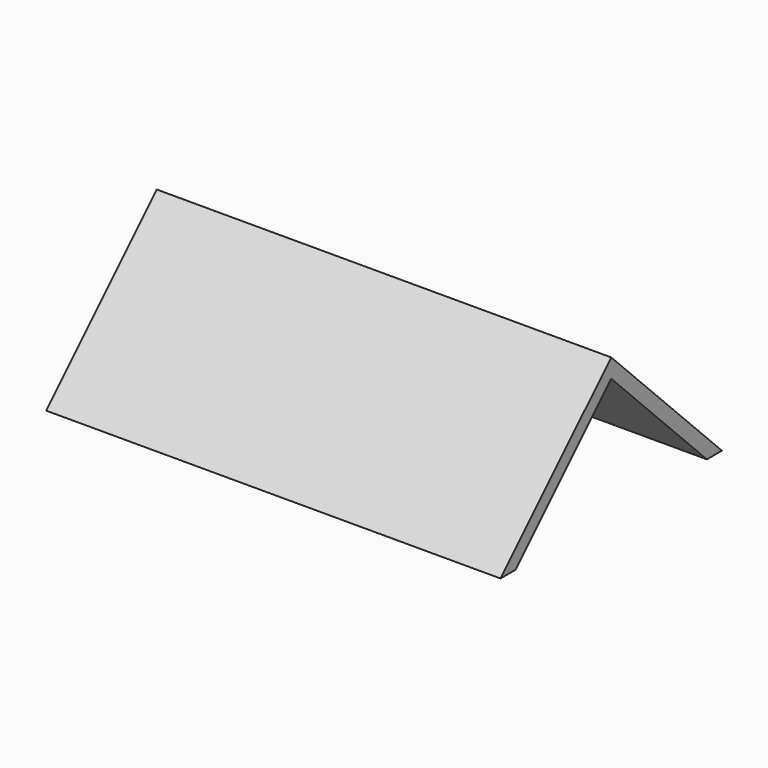
from build123d import *

# Parameters (mm, degrees)
F1_DEPTH = 60
F2_DEPTH = 8.4


with BuildPart() as f1:
    # F0 (on Right) → F1 (new body)
    with BuildSketch(Plane.YZ):
        Polygon((-124.5425649285, 38.5748143829), (-106.5425649285, 56.5748143829), (-88.5425649285, 38.5748143829), (-85.7141378038, 38.5748143829), (-87.1283513662, 39.9890279453), (-106.5425649285, 59.4032415077), (-125.9567784909, 39.9890279453), (-127.3709920533, 38.5748143829), align=None)
    extrude(amount=F1_DEPTH)

    # F2 (add): a face of the model
    f2_faces = [f1.faces().sort_by_distance(p)[0] for p in [
        (0, -125.9567784909, 39.0405521721),
    ]]
    extrude(f2_faces, amount=F2_DEPTH)


solid = f1.part
